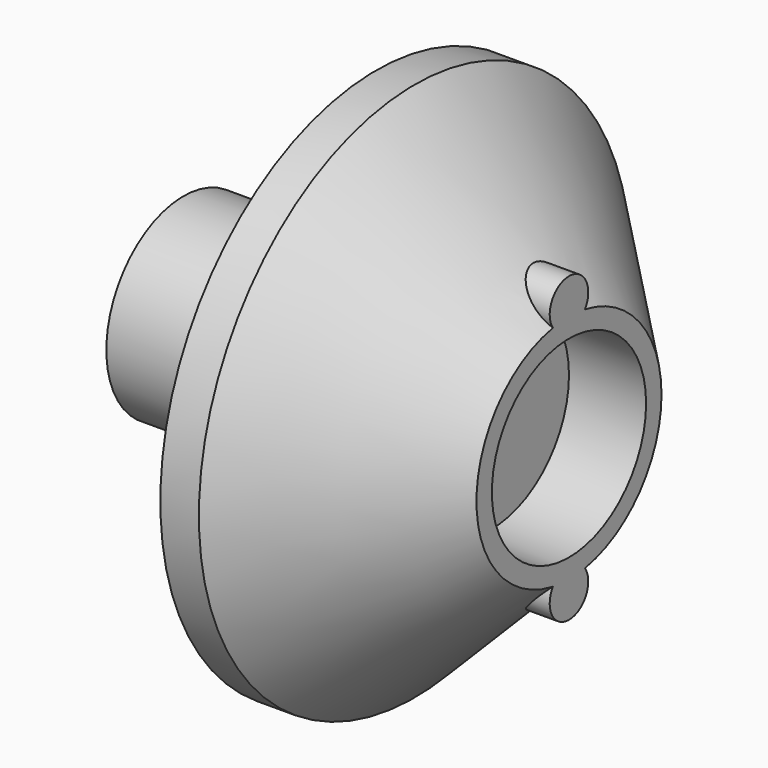
from build123d import *

# Parameters (mm, degrees)
F0_R     = 17.78
F0_R_2   = 1.5875
F0_R_3   = 6.35
F1_DEPTH = 12.7
F3_DEPTH = 7.62
F4_DEPTH = 12.7
F5_DEPTH = 12.7


# Not quite as in the source:
# - a fillet or chamfer that OpenCascade refuses, or shapes differently, is made with other operations: its cross-section is extruded or revolved along the edge and cut away or added


with BuildPart() as f1:
    # F0 (on Right) → F1 (new body)
    with BuildSketch(Plane.YZ):
        Circle(F0_R)
        with Locations((0, -8.382)):
            Circle(F0_R_2, mode=Mode.SUBTRACT)
        Circle(F0_R_3, mode=Mode.SUBTRACT)
        with Locations((0, 8.382)):
            Circle(F0_R_2, mode=Mode.SUBTRACT)
    extrude(amount=F1_DEPTH)

    # F2: chamfer of 10.16 on 1 edges, made by hand

    # F2_s1 → F2_t2 (revolve, cut)
    with BuildSketch(Plane.XY):
        Polygon((2.54, 17.78), (12.7, 7.62), (12.7, 17.78), align=None)
    revolve(axis=Axis((12.7, 0, 0), (1, 0, 0)), mode=Mode.SUBTRACT)

    # F0 (on Right) → F3 (join)
    with BuildSketch(Plane.YZ):
        Circle(F0_R_3)
    extrude(amount=F3_DEPTH)

    # F0 (on Right) → F4 (join)
    with BuildSketch(Plane.YZ):
        with Locations((0, 8.382)):
            Circle(F0_R_2)
        with Locations((0, -8.382)):
            Circle(F0_R_2)
    extrude(amount=F4_DEPTH)

    # F0 (on Right) → F5 (join)
    with BuildSketch(Plane.YZ):
        Circle(F0_R_3)
    extrude(amount=-F5_DEPTH)


solid = f1.part
